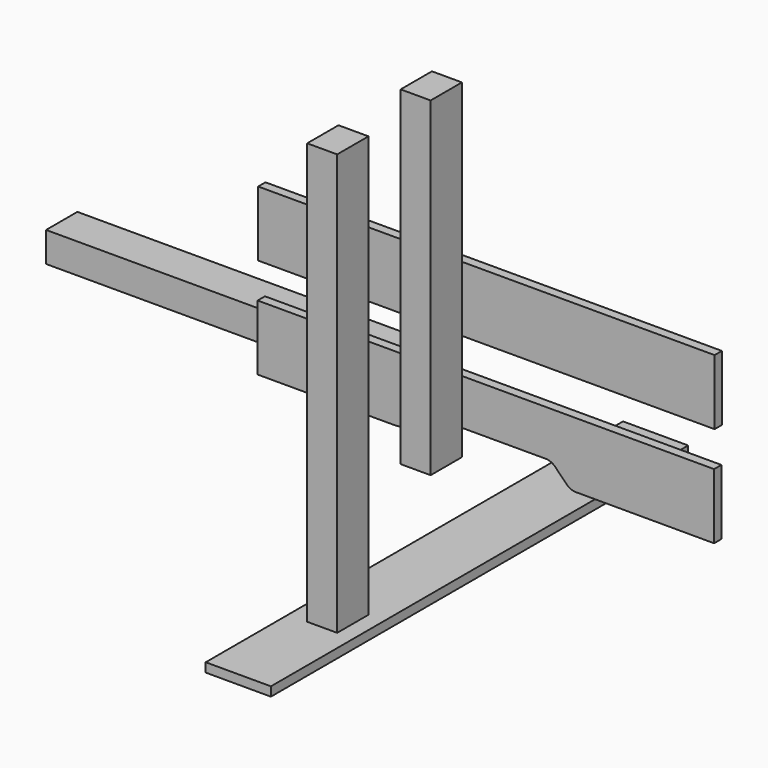
from build123d import *

# Parameters (mm, degrees)
F0_W     = 50
F0_H     = 400
F1_DEPTH = 7
F2_W     = 350
F2_H     = 50
F3_DEPTH = 7
F4_W     = 290
F4_H     = 30
F5_DEPTH = 23
F6_W     = 30
F6_H     = 253
F7_DEPTH = 23
F6_H_2   = 323


# Not quite as in the source:
# - a feature names something its author has since deleted; it is built from what else it names


with BuildPart() as f1:
    # F0 (on Top) → F1 (new body)
    with BuildSketch(Plane.XY):
        with Locations((-11.8191692954, 1.4386259147)):
            Rectangle(F0_W, F0_H)
    extrude(amount=F1_DEPTH)


with BuildPart() as f3:
    # F2 (on Front) → F3 (new body)
    with BuildSketch(Plane.XZ):
        with Locations((25.1859198511, 188.5405542329)):
            Rectangle(F2_W, F2_H)
    extrude(amount=F3_DEPTH)


with BuildPart() as f3b:
    # F2 (on Front) → F3, piece 2 (new body)
    with BuildSketch(Plane.XZ):
        with BuildLine():
            Line((199.7836618459, 136.4482086897), (-150.2163381541, 136.4482086897))
            Line((-150.2163381541, 136.4482086897), (-150.2163381541, 86.4482086897))
            Line((-150.2163381541, 86.4482086897), (-44.2547228372, 86.4482086897))
            ThreePointArc((-44.2547228372, 86.4482086897), (-40.4278885136, 87.2094133646), (-37.1836550254, 89.3771408778))
            Line((-37.1836550254, 89.3771408778), (-28.0415194017, 98.5192765016))
            ThreePointArc((-28.0415194017, 98.5192765016), (-24.7972859134, 100.6870040148), (-20.9704515898, 101.4482086897))
            Line((-20.9704515898, 101.4482086897), (70.6951992973, 101.4482086897))
            ThreePointArc((70.6951992973, 101.4482086897), (74.5614190603, 100.6705915024), (77.8263510358, 98.4586776385))
            Line((77.8263510358, 98.4586776385), (86.697224144, 89.4350955287))
            ThreePointArc((86.697224144, 89.4350955287), (89.9592474476, 87.2244015816), (93.8220676124, 86.4455664673))
            Line((93.8220676124, 86.4455664673), (199.7836618459, 86.3787230186))
            Line((199.7836618459, 86.3787230186), (199.7836618459, 136.4482086897))
        make_face()
    extrude(amount=F3_DEPTH)


with BuildPart() as f5:
    # F4 (on Top) → F5 (new body)
    with BuildSketch(Plane.XY):
        with Locations((-297.4768000841, 170.5034965277)):
            Rectangle(F4_W, F4_H)
    extrude(amount=F5_DEPTH)


with BuildPart() as f7:
    # F6 (on Right) → F7 (new body)
    with BuildSketch(Plane.YZ):
        with Locations((-42.7408777177, 221.9668109119)):
            Rectangle(F6_W, F6_H)
    extrude(amount=F7_DEPTH)


with BuildPart() as f7b:
    # F6 (on Right) → F7, piece 2 (new body)
    with BuildSketch(Plane.YZ):
        with Locations((-132.3216563463, 186.9668109119)):
            Rectangle(F6_W, F6_H_2)
    extrude(amount=F7_DEPTH)


solid = Compound([f1.part, f3.part, f3b.part, f5.part, f7.part, f7b.part])
